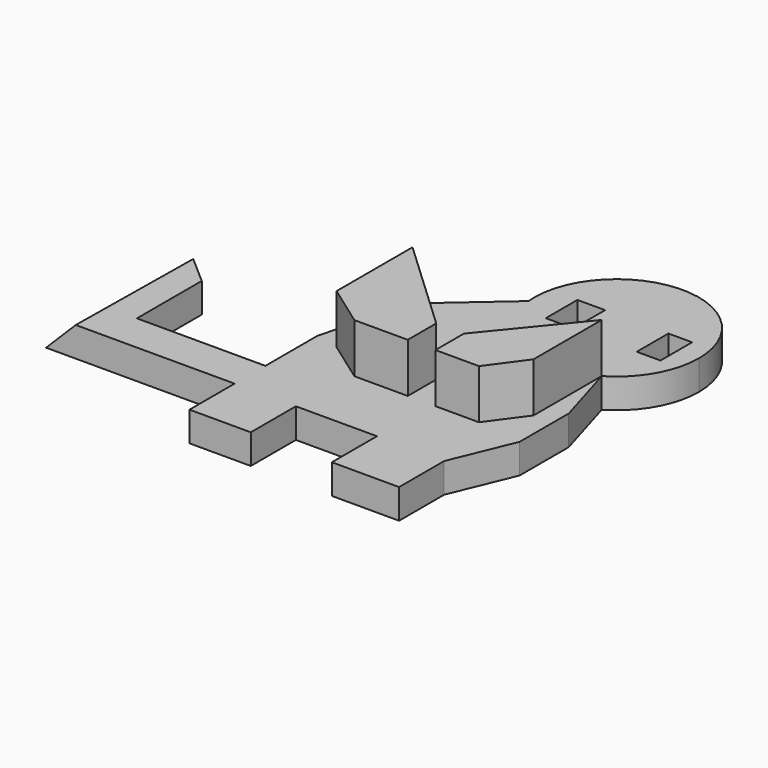
from build123d import *

# Parameters (mm, degrees)
F0_W        = 4.267198965
F0_H        = 6.0959979892
F0_W_2      = 3.6575980484
F1_DEPTH    = 4.572
F3_DEPTH    = 7.62
F4_T1_DEPTH = 48.8379448434


# Not quite as in the source:
# - a fillet or chamfer that OpenCascade refuses, or shapes differently, is made with other operations: its cross-section is extruded or revolved along the edge and cut away or added


with BuildPart() as f1:
    # F0 (on Top) → F1 (new body)
    with BuildSketch(Plane.XY):
        Polygon((0, 0), (0, 5.9436000884), (-19.8120009154, 5.9436000884), (-19.8120009154, 18.4403993189), (-24.6888007969, 22.7076001465), (-29.2608011514, 22.7076001465), (-29.5656006783, 0), align=None)
        with BuildLine():
            ThreePointArc((33.2821442915, 29.1467721924), (37.8525571162, 33.7863108871), (39.522399348, 40.0811992586))
            ThreePointArc((39.522399348, 40.0811992586), (26.2356214248, 52.7676365705), (14.1766211325, 38.9088966856))
            ThreePointArc((14.1766211325, 38.9088966856), (21.0438596912, 28.7719782671), (33.2821442915, 29.1467721924))
        make_face()
        with Locations((20.7264004275, 39.7763997316)):
            Rectangle(F0_W, F0_H, mode=Mode.SUBTRACT)
        with Locations((34.4424042851, 39.7763997316)):
            Rectangle(F0_W_2, F0_H, mode=Mode.SUBTRACT)
        with BuildLine():
            ThreePointArc((33.2821442915, 29.1467721924), (21.0438596912, 28.7719782671), (14.1766211325, 38.9088966856))
            Line((14.1766211325, 38.9088966856), (3.6576006096, 29.7180004418))
            Line((3.6576006096, 29.7180004418), (0, 16.0020012408))
            Line((0, 16.0020012408), (0, 5.9436000884))
            Line((0, 5.9436000884), (0, 0))
            Line((0, 0), (0, -8.686799556))
            Line((0, -8.686799556), (9.4487993047, -8.686799556))
            Line((9.4487993047, -8.686799556), (9.4487993047, 0))
            Line((9.4487993047, 0), (21.9455994666, 0))
            Line((21.9455994666, 0), (21.9455994666, -8.686799556))
            Line((21.9455994666, -8.686799556), (32.3087982833, -8.686799556))
            Line((32.3087982833, -8.686799556), (32.3087982833, 0))
            Line((32.3087982833, 0), (36.2712033093, 9.6011999995))
            Line((36.2712033093, 9.6011999995), (36.2712033093, 19.0500002354))
            Line((36.2712033093, 19.0500002354), (33.2821442915, 29.1467721924))
        make_face()
        Polygon((3.6576006096, 15.6971998513), (3.6576006096, 29.7180004418), (19.2023999989, 15.6971998513), (19.2023999989, 9.9060004577), (11.8871992454, 9.9060004577), align=None, mode=Mode.SUBTRACT)
        Polygon((23.7743984908, 14.3256001174), (33.2821442915, 29.1467721924), (32.6136052608, 14.3256001174), (28.0415974557, 9.6011999995), (23.7743984908, 9.6011999995), align=None, mode=Mode.SUBTRACT)
        Polygon((19.2023999989, 15.6971998513), (3.6576006096, 29.7180004418), (3.6576006096, 15.6971998513), (11.8871992454, 9.9060004577), (19.2023999989, 9.9060004577), align=None)
        Polygon((32.6136052608, 14.3256001174), (33.2821442915, 29.1467721924), (23.7743984908, 14.3256001174), (23.7743984908, 9.6011999995), (28.0415974557, 9.6011999995), align=None)
    extrude(amount=F1_DEPTH)

    # F2 (on face) → F3 (join)
    with BuildSketch(Plane.XY.offset(4.572)):
        Polygon((18.2879995555, 16.0020012408), (3.6576006096, 29.7180004418), (3.6576006096, 15.0875998661), (10.0584011525, 10.5156004429), (18.2879995555, 10.5156004429), align=None)
        Polygon((33.2821442915, 16.0020012408), (33.2821442915, 29.1467721924), (22.5551985204, 16.0020012408), (22.5551985204, 10.5156004429), (29.260803014, 10.5156004429), align=None)
    extrude(amount=F3_DEPTH)

    # F4: chamfer of 5.08 on 1 edges, made by hand

    # F4_s2 → F4_t1 (cut)
    with BuildSketch(Plane(origin=(0.4748152519, 35.3737913975, 0), x_dir=(0, 0, 1), z_dir=(-0.0134215888, -0.9999099264, 0))):
        Polygon((4.572, 24.4829375988), (-0.508, 29.5629375988), (4.572, 29.5629375988), align=None)
    extrude(amount=F4_T1_DEPTH, mode=Mode.SUBTRACT)


solid = f1.part
